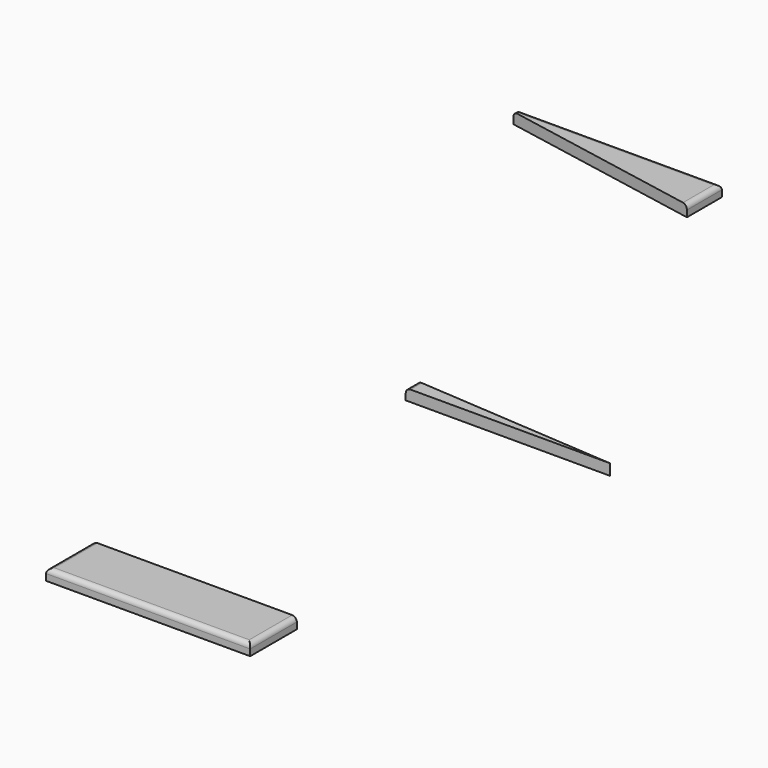
from build123d import *

# Parameters (mm, degrees)
F0_W     = 350
F0_H     = 100
F3_DEPTH = 19
F4_DEPTH = 19
F5_DEPTH = 19
F6_R     = 8
F6_2_R   = 8
F6_3_R   = 8


# Not quite as in the source:
# - a feature names something its author has since deleted; it is built from what else it names


with BuildPart() as f3:
    # F0 (on Top) → F3 (new body)
    with BuildSketch(Plane.XY):
        with Locations((-4547.6745605469, -3248.0629263303)):
            Rectangle(F0_W, F0_H)
    extrude(amount=F3_DEPTH)

    # F6#3
    f6_3_edges = [f3.edges().sort_by_distance(p)[0] for p in [
        (-4722.674561, -3248.062926, 19),
        (-4372.674561, -3248.062926, 19),
        (-4547.674561, -3298.062926, 19),
    ]]
    fillet(f6_3_edges, radius=F6_3_R)


with BuildPart() as f4:
    # F1 (on Top) → F4 (new body)
    with BuildSketch(Plane.XY):
        Polygon((-4711.1567020416, -1863.7687733282), (-5061.1567020416, -1863.7687733282), (-5061.1567020416, -1873.1437733282), (-4711.1567020416, -1938.7687733282), align=None)
    extrude(amount=F4_DEPTH)

    # F6
    f6_edges = [f4.edges().sort_by_distance(p)[0] for p in [
        (-5061.156702, -1868.456273, 19),
        (-4886.156702, -1863.768773, 19),
        (-4711.156702, -1901.268773, 19),
    ]]
    fillet(f6_edges, radius=F6_R)


with BuildPart() as f5:
    # F2 (on Top) → F5 (new body)
    with BuildSketch(Plane.XY):
        Polygon((-4673.5225359599, -2563.5657919492), (-4673.5225359599, -2588.5657919492), (-4323.5225359599, -2588.5657919492), align=None)
    extrude(amount=F5_DEPTH)

    # F6#2
    f6_2_edges = [f5.edges().sort_by_distance(p)[0] for p in [
        (-4673.522536, -2576.065792, 19),
    ]]
    fillet(f6_2_edges, radius=F6_2_R)


solid = Compound([f3.part, f4.part, f5.part])
